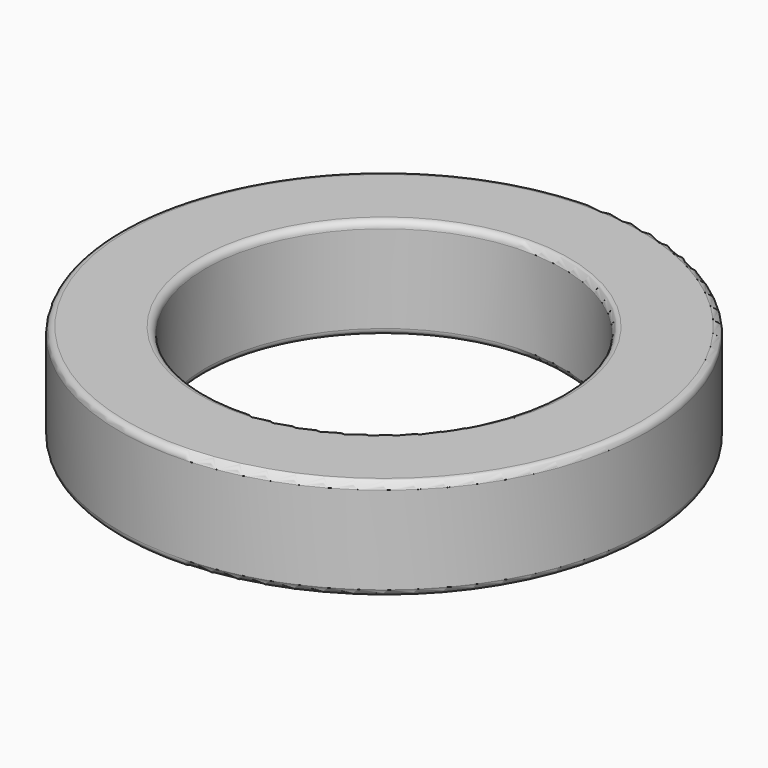
from build123d import *

# Parameters (mm, degrees)
F0_R     = 193.1582177029
F0_R_2   = 191.8011573182
F0_R_3   = 130.4635260733
F1_DEPTH = 74.2441564798
F5_R     = 5


# Not quite as in the source:
# - the program builds the solid bodies; features that only make, move or delete a surface that nothing else refers to are left out


with BuildPart() as f1:
    # F0 (on Top) → F1 (new body)
    with BuildSketch(Plane.XY):
        Circle(F0_R)
        Circle(F0_R_2, mode=Mode.SUBTRACT)
        Circle(F0_R_2)
        Circle(F0_R_3, mode=Mode.SUBTRACT)
    extrude(amount=F1_DEPTH)

    # F5
    f5_edges = [f1.edges().sort_by_distance(p)[0] for p in [
        (-193.158218, 0, 74.244156),
        (-130.463526, 0, 0),
        (-193.158218, 0, 0),
        (-130.463526, 0, 74.244156),
    ]]
    fillet(f5_edges, radius=F5_R)


solid = f1.part
